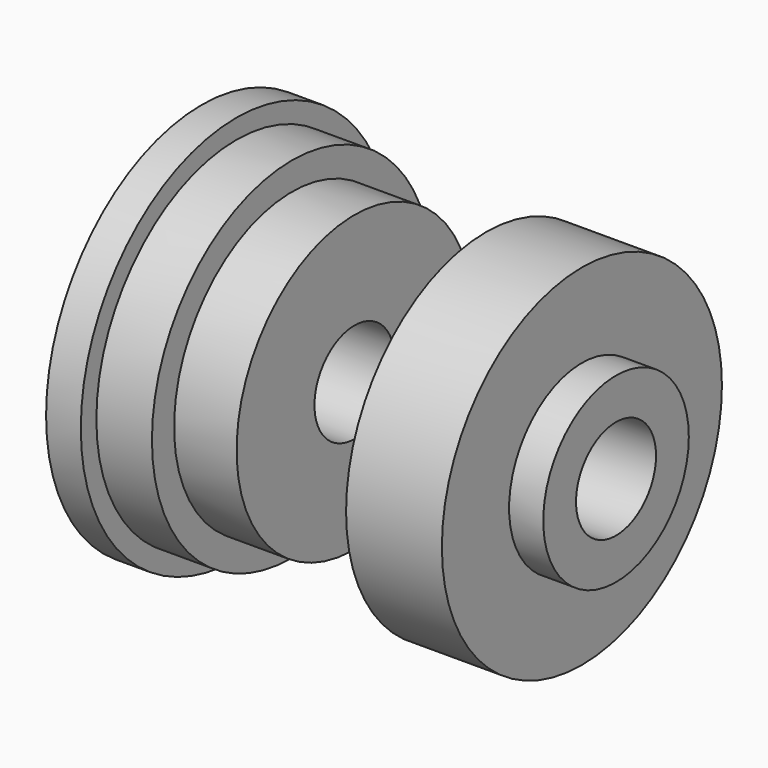
from build123d import *

# Parameters (mm, degrees)
F3_SIZE = 35


with BuildPart() as f1:
    # F0 (on Top) → F1 (revolve)
    with BuildSketch(Plane.XY):
        Polygon((-53.757738322, 162.981180191), (-53.757738322, 58.981180191), (56.242261678, 58.981180191), (56.242261678, 109.081180191), (56.242261678, 129.031180191), (11.242261678, 129.031180191), (11.242261678, 148.981180191), (-28.757738322, 148.981180191), (-28.757738322, 162.981180191), align=None)
    revolve(axis=Axis((-73.0837285519, 22.981180191, 0), (1, 0, 0)))

    # F3
    f3_edges = [f1.edges().sort_by_distance(p)[0] for p in [
        (-53.757738, -13.01882, 0),
    ]]
    chamfer(f3_edges, length=F3_SIZE)


with BuildPart() as f2:
    # F0 (on Top) → F2 (revolve)
    with BuildSketch(Plane.XY):
        Polygon((195.9919762611, 128.981180191), (195.9919762611, 58.981180191), (219.9965119362, 58.981180191), (244.5349097252, 58.981180191), (244.5349097252, 88.4826818109), (219.966635108, 88.4826818109), (219.966635108, 128.981180191), align=None)
        Polygon((150.9919762611, 128.981180191), (195.9919762611, 128.981180191), (219.966635108, 128.981180191), (219.966635108, 148.981180191), (150.9919762611, 148.981180191), align=None)
    revolve(axis=Axis((56.242261678, 22.981180191, 0), (1, 0, 0)))


solid = Compound([f1.part, f2.part])
